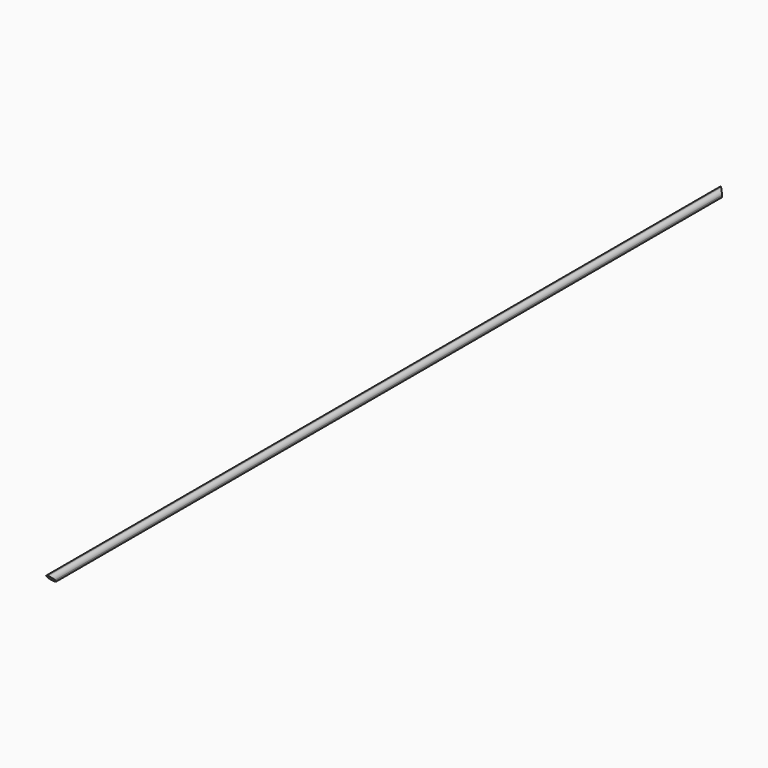
from build123d import *

# Parameters (mm, degrees)
F0_W     = 42
F0_H     = 42
F1_DEPTH = 4441
F3_DEPTH = 100
F5_DEPTH = 100
F6_R     = 20.99999


# Not quite as in the source:
# - a fillet or chamfer is up to 0.001 mm smaller than in the source, because OpenCascade refuses the exact size


with BuildPart() as f1:
    # F0 (on Front) → F1 (new body)
    with BuildSketch(Plane.XZ):
        Rectangle(F0_W, F0_H)
    extrude(amount=F1_DEPTH)

    # F2 (on face) → F3 (cut)
    with BuildSketch(Plane.YZ.offset(21)):
        Polygon((-4399, -21), (-4441, 21), (-4441, -21), align=None)
    extrude(amount=-F3_DEPTH, mode=Mode.SUBTRACT)

    # F4 (on face) → F5 (cut)
    with BuildSketch(Plane(origin=(0, 0, -21), x_dir=(1, 0, 0), z_dir=(0, 0, -1))):
        Polygon((21, 42), (-21, 0), (21, 0), align=None)
    extrude(amount=-F5_DEPTH, mode=Mode.SUBTRACT)

    # F6 (radius 21 in the source; OpenCascade refuses exactly that, so slightly less here)
    f6_edges = [f1.edges().sort_by_distance(p)[0] for p in [
        (-21, -2199.5, -21),
        (21, -2220.5, -21),
        (-21, -2220.5, 21),
        (21, -2241.5, 21),
    ]]
    fillet(f6_edges, radius=F6_R)


solid = f1.part
